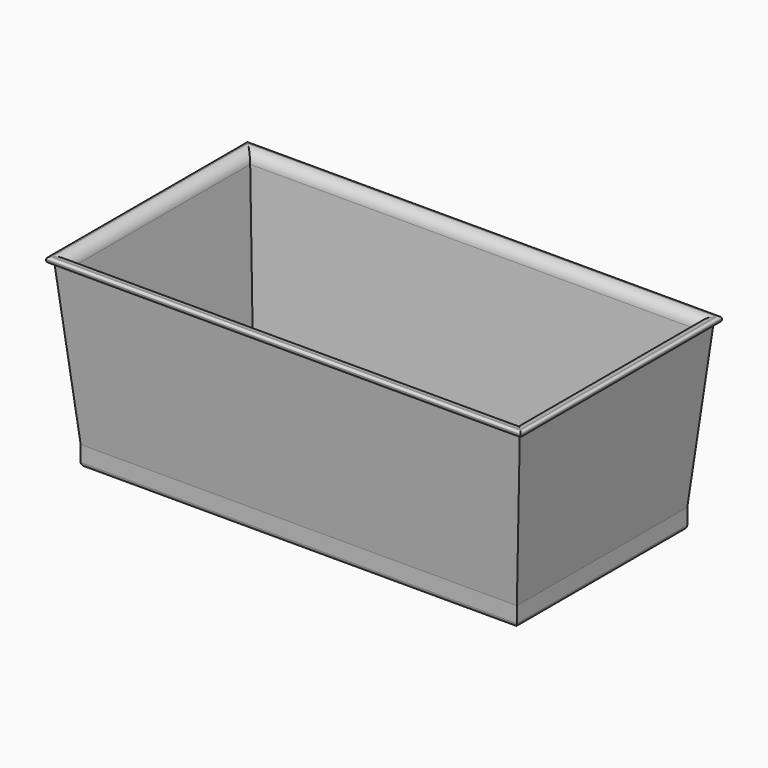
from build123d import *

# Parameters (mm, degrees)
F0_W         = 95.25
F0_H         = 44.45
F1_DEPTH     = 2.54
F4_T1_DEPTH  = 44.45
F4_T3_DEPTH  = 95.25
F4_T5_DEPTH  = 53.5988288205
F4_T7_DEPTH  = 104.3988288205
F4_T13_DEPTH = 46.9924144102
F4_T18_DEPTH = 97.7924144102
F4_T26_DEPTH = 46.9924144102
F4_T31_DEPTH = 97.7924144102
F4_T39_DEPTH = 97.7924144102
F4_T44_DEPTH = 46.9924144102
F4_T52_DEPTH = 46.9924144102
F4_T57_DEPTH = 97.7924144102
F5_R         = 5.08
F6_R         = 2.54
F7_R         = 0.508


# Not quite as in the source:
# - a fillet or chamfer that OpenCascade refuses, or shapes differently, is made with other operations: its cross-section is extruded or revolved along the edge and cut away or added


with BuildPart() as f1:
    # F0 (on Top) → F1 (new body)
    with BuildSketch(Plane.XY):
        Rectangle(F0_W, F0_H)
    extrude(amount=F1_DEPTH)

    # F3: sweep along a path in F3_path
    with BuildLine(Plane(origin=(-47.625, 22.225, 2.54), x_dir=(0, -1, 0), z_dir=(0, 0, -1))) as f3_path:
        Line((0, 0), (44.45, 0))
        Line((44.45, 0), (44.45, -95.25))
        Line((44.45, -95.25), (0, -95.25))
        Line((0, -95.25), (0, 0))
    # F2 (on face) → F3 (sweep)
    with BuildSketch(Plane.XZ.offset(22.225)):
        Polygon((-52.9928505421, 39.2721965909), (-49.657, 2.54), (-49.657, -2.032), (-47.625, -2.032), (-47.625, 0), (-47.625, 2.54), (-50.9456337987, 40.4950179973), (-54.0375709534, 40.4950179973), (-54.0375709534, 39.2721965909), align=None)
    sweep(path=f3_path.line, transition=Transition.RIGHT)

    # F4: fillet of radius 1.016 on 16 edges, made by hand

    # F4_s2 → F4_t1 (cut)
    with BuildSketch(Plane.XZ.offset(-22.225)):
        with BuildLine():
            ThreePointArc((47.6246, -1.0150343146), (47.9225795103, -1.7344204897), (48.6419656854, -2.0324))
            Line((48.6419656854, -2.0324), (48.6419656854, -2.1341365685))
            ThreePointArc((48.6419656854, -2.1341365685), (48.1334828427, -2.1337365685), (47.625, -2.1337365685))
            Line((47.625, -2.1337365685), (47.5232634315, -2.032))
            ThreePointArc((47.5232634315, -2.032), (47.5232634315, -1.5235171573), (47.5228634315, -1.0150343146))
            Line((47.5228634315, -1.0150343146), (47.6246, -1.0150343146))
        make_face()
        with BuildLine():
            ThreePointArc((-47.6246, -1.0150343146), (-47.9225795103, -1.7344204897), (-48.6419656854, -2.0324))
            Line((-48.6419656854, -2.0324), (-48.6419656854, -2.1341365685))
            ThreePointArc((-48.6419656854, -2.1341365685), (-48.1334828427, -2.1337365685), (-47.625, -2.1337365685))
            Line((-47.625, -2.1337365685), (-47.5232634315, -2.032))
            ThreePointArc((-47.5232634315, -2.032), (-47.5232634315, -1.5235171573), (-47.5228634315, -1.0150343146))
            Line((-47.5228634315, -1.0150343146), (-47.6246, -1.0150343146))
        make_face()
    extrude(amount=F4_T1_DEPTH, mode=Mode.SUBTRACT)

    # F4_s4 → F4_t3 (cut)
    with BuildSketch(Plane.YZ.offset(-47.625)):
        with BuildLine():
            ThreePointArc((22.2246, -1.0150343146), (22.5225795103, -1.7344204897), (23.2419656854, -2.0324))
            Line((23.2419656854, -2.0324), (23.2419656854, -2.1341365685))
            ThreePointArc((23.2419656854, -2.1341365685), (22.7334828427, -2.1337365685), (22.225, -2.1337365685))
            Line((22.225, -2.1337365685), (22.1232634315, -2.032))
            ThreePointArc((22.1232634315, -2.032), (22.1232634315, -1.5235171573), (22.1228634315, -1.0150343146))
            Line((22.1228634315, -1.0150343146), (22.2246, -1.0150343146))
        make_face()
        with BuildLine():
            ThreePointArc((-22.2246, -1.0150343146), (-22.5225795103, -1.7344204897), (-23.2419656854, -2.0324))
            Line((-23.2419656854, -2.0324), (-23.2419656854, -2.1341365685))
            ThreePointArc((-23.2419656854, -2.1341365685), (-22.7334828427, -2.1337365685), (-22.225, -2.1337365685))
            Line((-22.225, -2.1337365685), (-22.1232634315, -2.032))
            ThreePointArc((-22.1232634315, -2.032), (-22.1232634315, -1.5235171573), (-22.1228634315, -1.0150343146))
            Line((-22.1228634315, -1.0150343146), (-22.2246, -1.0150343146))
        make_face()
    extrude(amount=F4_T3_DEPTH, mode=Mode.SUBTRACT)

    # F4_s6 → F4_t5 (cut)
    with BuildSketch(Plane.XZ.offset(-26.7994144102)):
        with BuildLine():
            ThreePointArc((-48.6400343146, -2.0324), (-49.3594204897, -1.7344204897), (-49.6574, -1.0150343146))
            Line((-49.6574, -1.0150343146), (-49.7591365685, -1.0150343146))
            ThreePointArc((-49.7591365685, -1.0150343146), (-49.7587365685, -1.5235171573), (-49.7587365685, -2.032))
            Line((-49.7587365685, -2.032), (-49.657, -2.1337365685))
            ThreePointArc((-49.657, -2.1337365685), (-49.1485171573, -2.1337365685), (-48.6400343146, -2.1341365685))
            Line((-48.6400343146, -2.1341365685), (-48.6400343146, -2.0324))
        make_face()
        with BuildLine():
            ThreePointArc((48.6400343146, -2.0324), (49.3594204897, -1.7344204897), (49.6574, -1.0150343146))
            Line((49.6574, -1.0150343146), (49.7591365685, -1.0150343146))
            ThreePointArc((49.7591365685, -1.0150343146), (49.7587365685, -1.5235171573), (49.7587365685, -2.032))
            Line((49.7587365685, -2.032), (49.657, -2.1337365685))
            ThreePointArc((49.657, -2.1337365685), (49.1485171573, -2.1337365685), (48.6400343146, -2.1341365685))
            Line((48.6400343146, -2.1341365685), (48.6400343146, -2.0324))
        make_face()
    extrude(amount=F4_T5_DEPTH, mode=Mode.SUBTRACT)

    # F4_s8 → F4_t7 (cut)
    with BuildSketch(Plane.YZ.offset(-52.1994144102)):
        with BuildLine():
            ThreePointArc((23.2400343146, -2.0324), (23.9594204897, -1.7344204897), (24.2574, -1.0150343146))
            Line((24.2574, -1.0150343146), (24.3591365685, -1.0150343146))
            ThreePointArc((24.3591365685, -1.0150343146), (24.3587365685, -1.5235171573), (24.3587365685, -2.032))
            Line((24.3587365685, -2.032), (24.257, -2.1337365685))
            ThreePointArc((24.257, -2.1337365685), (23.7485171573, -2.1337365685), (23.2400343146, -2.1341365685))
            Line((23.2400343146, -2.1341365685), (23.2400343146, -2.0324))
        make_face()
        with BuildLine():
            ThreePointArc((-23.2400343146, -2.0324), (-23.9594204897, -1.7344204897), (-24.2574, -1.0150343146))
            Line((-24.2574, -1.0150343146), (-24.3591365685, -1.0150343146))
            ThreePointArc((-24.3591365685, -1.0150343146), (-24.3587365685, -1.5235171573), (-24.3587365685, -2.032))
            Line((-24.3587365685, -2.032), (-24.257, -2.1337365685))
            ThreePointArc((-24.257, -2.1337365685), (-23.7485171573, -2.1337365685), (-23.2400343146, -2.1341365685))
            Line((-23.2400343146, -2.1341365685), (-23.2400343146, -2.0324))
        make_face()
    extrude(amount=F4_T7_DEPTH, mode=Mode.SUBTRACT)


with BuildPart() as f4_tool11:
    # F4_s12 → F4_t13 (new body)
    with BuildSketch(Plane.XZ.offset(24.7674144102)):
        with BuildLine():
            ThreePointArc((47.6246, -1.0150343146), (47.9225795103, -1.7344204897), (48.6419656854, -2.0324))
            Line((48.6419656854, -2.0324), (48.6419656854, -2.1341365685))
            ThreePointArc((48.6419656854, -2.1341365685), (48.1334828427, -2.1337365685), (47.625, -2.1337365685))
            Line((47.625, -2.1337365685), (47.5232634315, -2.032))
            ThreePointArc((47.5232634315, -2.032), (47.5232634315, -1.5235171573), (47.5228634315, -1.0150343146))
            Line((47.5228634315, -1.0150343146), (47.6246, -1.0150343146))
        make_face()
    extrude(amount=-F4_T13_DEPTH)

    split(bisect_by=Plane.XZ.offset(22.225), keep=Keep.TOP)

    split(bisect_by=Plane.XZ.offset(24.257), keep=Keep.BOTTOM)


with BuildPart() as f4_tool16:
    # F4_s17 → F4_t18 (new body)
    with BuildSketch(Plane.YZ.offset(-47.625)):
        with BuildLine():
            ThreePointArc((-22.2246, -1.0150343146), (-22.5225795103, -1.7344204897), (-23.2419656854, -2.0324))
            Line((-23.2419656854, -2.0324), (-23.2419656854, -2.1341365685))
            ThreePointArc((-23.2419656854, -2.1341365685), (-22.7334828427, -2.1337365685), (-22.225, -2.1337365685))
            Line((-22.225, -2.1337365685), (-22.1232634315, -2.032))
            ThreePointArc((-22.1232634315, -2.032), (-22.1232634315, -1.5235171573), (-22.1228634315, -1.0150343146))
            Line((-22.1228634315, -1.0150343146), (-22.2246, -1.0150343146))
        make_face()
    extrude(amount=F4_T18_DEPTH)

    split(bisect_by=Plane.YZ.offset(47.625), keep=Keep.TOP)

    split(bisect_by=Plane.YZ.offset(49.657), keep=Keep.BOTTOM)


with BuildPart() as f4_tool11_1:
    add(f4_tool11.part)

    # F4_t21: intersect F4_tool16
    add(f4_tool16.part, mode=Mode.INTERSECT)


with BuildPart() as f1_1:
    add(f1.part)

    # F4_t9: cut F4_tool11
    add(f4_tool11_1.part, mode=Mode.SUBTRACT)


with BuildPart() as f4_tool24:
    # F4_s25 → F4_t26 (new body)
    with BuildSketch(Plane.XZ.offset(22.225)):
        with BuildLine():
            ThreePointArc((47.6246, -1.0150343146), (47.9225795103, -1.7344204897), (48.6419656854, -2.0324))
            Line((48.6419656854, -2.0324), (48.6419656854, -2.1341365685))
            ThreePointArc((48.6419656854, -2.1341365685), (48.1334828427, -2.1337365685), (47.625, -2.1337365685))
            Line((47.625, -2.1337365685), (47.5232634315, -2.032))
            ThreePointArc((47.5232634315, -2.032), (47.5232634315, -1.5235171573), (47.5228634315, -1.0150343146))
            Line((47.5228634315, -1.0150343146), (47.6246, -1.0150343146))
        make_face()
    extrude(amount=-F4_T26_DEPTH)

    split(bisect_by=Plane.XZ.offset(-22.225), keep=Keep.BOTTOM)

    split(bisect_by=Plane.XZ.offset(-24.257), keep=Keep.TOP)


with BuildPart() as f4_tool29:
    # F4_s30 → F4_t31 (new body)
    with BuildSketch(Plane.YZ.offset(50.1674144102)):
        with BuildLine():
            ThreePointArc((22.2246, -1.0150343146), (22.5225795103, -1.7344204897), (23.2419656854, -2.0324))
            Line((23.2419656854, -2.0324), (23.2419656854, -2.1341365685))
            ThreePointArc((23.2419656854, -2.1341365685), (22.7334828427, -2.1337365685), (22.225, -2.1337365685))
            Line((22.225, -2.1337365685), (22.1232634315, -2.032))
            ThreePointArc((22.1232634315, -2.032), (22.1232634315, -1.5235171573), (22.1228634315, -1.0150343146))
            Line((22.1228634315, -1.0150343146), (22.2246, -1.0150343146))
        make_face()
    extrude(amount=-F4_T31_DEPTH)

    split(bisect_by=Plane.YZ.offset(47.625), keep=Keep.TOP)

    split(bisect_by=Plane.YZ.offset(49.657), keep=Keep.BOTTOM)


with BuildPart() as f4_tool24_1:
    add(f4_tool24.part)

    # F4_t34: intersect F4_tool29
    add(f4_tool29.part, mode=Mode.INTERSECT)


with BuildPart() as f1_2:
    add(f1_1.part)

    # F4_t22: cut F4_tool24
    add(f4_tool24_1.part, mode=Mode.SUBTRACT)


with BuildPart() as f4_tool37:
    # F4_s38 → F4_t39 (new body)
    with BuildSketch(Plane.YZ.offset(47.625)):
        with BuildLine():
            ThreePointArc((22.2246, -1.0150343146), (22.5225795103, -1.7344204897), (23.2419656854, -2.0324))
            Line((23.2419656854, -2.0324), (23.2419656854, -2.1341365685))
            ThreePointArc((23.2419656854, -2.1341365685), (22.7334828427, -2.1337365685), (22.225, -2.1337365685))
            Line((22.225, -2.1337365685), (22.1232634315, -2.032))
            ThreePointArc((22.1232634315, -2.032), (22.1232634315, -1.5235171573), (22.1228634315, -1.0150343146))
            Line((22.1228634315, -1.0150343146), (22.2246, -1.0150343146))
        make_face()
    extrude(amount=-F4_T39_DEPTH)

    split(bisect_by=Plane.YZ.offset(-47.625), keep=Keep.BOTTOM)

    split(bisect_by=Plane.YZ.offset(-49.657), keep=Keep.TOP)


with BuildPart() as f4_tool42:
    # F4_s43 → F4_t44 (new body)
    with BuildSketch(Plane.XZ.offset(-24.7674144102)):
        with BuildLine():
            ThreePointArc((-47.6246, -1.0150343146), (-47.9225795103, -1.7344204897), (-48.6419656854, -2.0324))
            Line((-48.6419656854, -2.0324), (-48.6419656854, -2.1341365685))
            ThreePointArc((-48.6419656854, -2.1341365685), (-48.1334828427, -2.1337365685), (-47.625, -2.1337365685))
            Line((-47.625, -2.1337365685), (-47.5232634315, -2.032))
            ThreePointArc((-47.5232634315, -2.032), (-47.5232634315, -1.5235171573), (-47.5228634315, -1.0150343146))
            Line((-47.5228634315, -1.0150343146), (-47.6246, -1.0150343146))
        make_face()
    extrude(amount=F4_T44_DEPTH)

    split(bisect_by=Plane.XZ.offset(-22.225), keep=Keep.BOTTOM)

    split(bisect_by=Plane.XZ.offset(-24.257), keep=Keep.TOP)


with BuildPart() as f4_tool37_1:
    add(f4_tool37.part)

    # F4_t47: intersect F4_tool42
    add(f4_tool42.part, mode=Mode.INTERSECT)


with BuildPart() as f1_3:
    add(f1_2.part)

    # F4_t35: cut F4_tool37
    add(f4_tool37_1.part, mode=Mode.SUBTRACT)


with BuildPart() as f4_tool50:
    # F4_s51 → F4_t52 (new body)
    with BuildSketch(Plane.XZ.offset(-22.225)):
        with BuildLine():
            ThreePointArc((-47.6246, -1.0150343146), (-47.9225795103, -1.7344204897), (-48.6419656854, -2.0324))
            Line((-48.6419656854, -2.0324), (-48.6419656854, -2.1341365685))
            ThreePointArc((-48.6419656854, -2.1341365685), (-48.1334828427, -2.1337365685), (-47.625, -2.1337365685))
            Line((-47.625, -2.1337365685), (-47.5232634315, -2.032))
            ThreePointArc((-47.5232634315, -2.032), (-47.5232634315, -1.5235171573), (-47.5228634315, -1.0150343146))
            Line((-47.5228634315, -1.0150343146), (-47.6246, -1.0150343146))
        make_face()
    extrude(amount=F4_T52_DEPTH)

    split(bisect_by=Plane.XZ.offset(22.225), keep=Keep.TOP)

    split(bisect_by=Plane.XZ.offset(24.257), keep=Keep.BOTTOM)


with BuildPart() as f4_tool55:
    # F4_s56 → F4_t57 (new body)
    with BuildSketch(Plane.YZ.offset(-50.1674144102)):
        with BuildLine():
            ThreePointArc((-22.2246, -1.0150343146), (-22.5225795103, -1.7344204897), (-23.2419656854, -2.0324))
            Line((-23.2419656854, -2.0324), (-23.2419656854, -2.1341365685))
            ThreePointArc((-23.2419656854, -2.1341365685), (-22.7334828427, -2.1337365685), (-22.225, -2.1337365685))
            Line((-22.225, -2.1337365685), (-22.1232634315, -2.032))
            ThreePointArc((-22.1232634315, -2.032), (-22.1232634315, -1.5235171573), (-22.1228634315, -1.0150343146))
            Line((-22.1228634315, -1.0150343146), (-22.2246, -1.0150343146))
        make_face()
    extrude(amount=F4_T57_DEPTH)

    split(bisect_by=Plane.YZ.offset(-47.625), keep=Keep.BOTTOM)

    split(bisect_by=Plane.YZ.offset(-49.657), keep=Keep.TOP)


with BuildPart() as f4_tool50_1:
    add(f4_tool50.part)

    # F4_t60: intersect F4_tool55
    add(f4_tool55.part, mode=Mode.INTERSECT)


with BuildPart() as f1_4:
    add(f1_3.part)

    # F4_t48: cut F4_tool50
    add(f4_tool50_1.part, mode=Mode.SUBTRACT)

    # F5
    f5_edges = [f1_4.edges().sort_by_distance(p)[0] for p in [
        (0, 22.225, 2.54),
        (-47.625, 0, 2.54),
        (47.625, 0, 2.54),
        (0, -22.225, 2.54),
    ]]
    fillet(f5_edges, radius=F5_R)

    # F6
    f6_edges = [f1_4.edges().sort_by_distance(p)[0] for p in [
        (0, -25.545634, 40.495018),
        (-50.945634, 0, 40.495018),
        (0, 25.545634, 40.495018),
        (50.945634, 0, 40.495018),
    ]]
    fillet(f6_edges, radius=F6_R)

    # F7
    f7_edges = [f1_4.edges().sort_by_distance(p)[0] for p in [
        (-54.037571, 0, 40.495018),
        (0, -28.637571, 40.495018),
        (54.037571, 0, 40.495018),
        (0, 28.637571, 40.495018),
        (-54.037571, 0, 39.272197),
        (0, -28.637571, 39.272197),
        (54.037571, 0, 39.272197),
        (0, 28.637571, 39.272197),
    ]]
    fillet(f7_edges, radius=F7_R)


solid = f1_4.part
